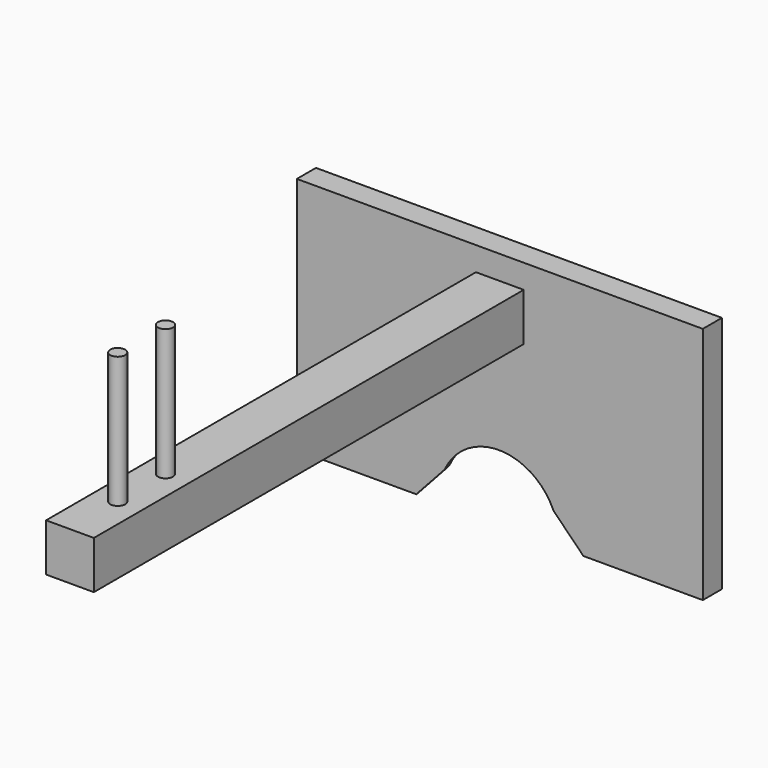
from build123d import *

# Parameters (mm, degrees)
F0_R     = 1.5875
F1_DEPTH = 10.16
F2_DEPTH = 38.1
F3_W     = 10.16
F3_H     = 10.16
F3_W_2   = 25.4
F3_H_2   = 50.8
F4_DEPTH = 5.08
F5_DEPTH = 3.81
F6_R     = 5.07999


# Not quite as in the source:
# - a fillet or chamfer is up to 0.001 mm smaller than in the source, because OpenCascade refuses the exact size
# - a feature names something its author has since deleted; it is built from what else it names


with BuildPart() as f1:
    # F0 (on Top) → F1 (new body)
    with BuildSketch(Plane.XY):
        Polygon((24.5562880617, 49.3353436351), (14.3962880617, 49.3353436351), (14.3962880617, -7.8146563649), (14.3962880617, -39.5646563649), (14.3962880617, -64.9646563649), (24.5562880617, -64.9646563649), align=None)
        with Locations((19.4762880617, -39.5646563649)):
            Circle(F0_R, mode=Mode.SUBTRACT)
        with Locations((19.4762880617, -52.2646563649)):
            Circle(F0_R, mode=Mode.SUBTRACT)
    extrude(amount=F1_DEPTH)

    # F0 (on Top) → F2 (join)
    with BuildSketch(Plane.XY):
        with Locations((19.4762880617, -39.5646563649)):
            Circle(F0_R)
        with Locations((19.4762880617, -52.2646563649)):
            Circle(F0_R)
    extrude(amount=F2_DEPTH)

    # F3 (on face) → F4 (join)
    with BuildSketch(Plane(origin=(0, 49.3353436351, 0), x_dir=(-1, 0, 0), z_dir=(0, 1, 0))):
        with BuildLine():
            Line((-24.5562880617, 0), (-24.5562880617, 10.16))
            Line((-24.5562880617, 10.16), (-24.5562880617, 15.24))
            Line((-24.5562880617, 15.24), (-37.2562880617, 15.24))
            Line((-37.2562880617, 15.24), (-37.2562880617, -35.56))
            Line((-37.2562880617, -35.56), (-30.9062880617, -29.15440273))
            ThreePointArc((-30.9062880617, -29.15440273), (-19.3773342754, -21.5585615124), (-7.7287880617, -28.9696984238))
            Line((-7.7287880617, -28.9696984238), (-1.6962880617, -35.56))
            Line((-1.6962880617, -35.56), (-1.6962880617, 10.16))
            Line((-1.6962880617, 10.16), (-14.3962880617, 10.16))
            Line((-14.3962880617, 10.16), (-14.3962880617, 0))
            Line((-14.3962880617, 0), (-24.5562880617, 0))
        make_face()
        Polygon((-24.5562880617, 15.24), (-24.5562880617, 10.16), (-14.3962880617, 10.16), (-1.6962880617, 10.16), (-1.6962880617, 15.24), (-13.7612880617, 15.24), align=None)
        with Locations((-19.4762880617, 5.08)):
            Rectangle(F3_W, F3_H)
        with Locations((-49.9562880617, -10.16)):
            Rectangle(F3_W_2, F3_H_2)
        Polygon((-1.6962880617, 15.24), (-1.6962880617, 10.16), (-1.6962880617, -35.56), (23.7037119383, -35.56), (23.7037119383, 15.24), align=None)
    extrude(amount=F4_DEPTH)

    # F3 (on face) → F5 (join)
    with BuildSketch(Plane(origin=(0, 49.3353436351, 0), x_dir=(-1, 0, 0), z_dir=(0, 1, 0))):
        with Locations((-19.4762880617, 5.08)):
            Rectangle(F3_W, F3_H)
    extrude(amount=F5_DEPTH)

    # F6 (radius 5.08 in the source; OpenCascade refuses exactly that, so slightly less here)
    f6_edges = [f1.edges().sort_by_distance(p)[0] for p in [
        (19.377334, 54.415344, -21.558562),
        (4.712538, 54.415344, -32.264849),
        (34.081288, 54.415344, -32.357201),
    ]]
    fillet(f6_edges, radius=F6_R)


solid = f1.part
